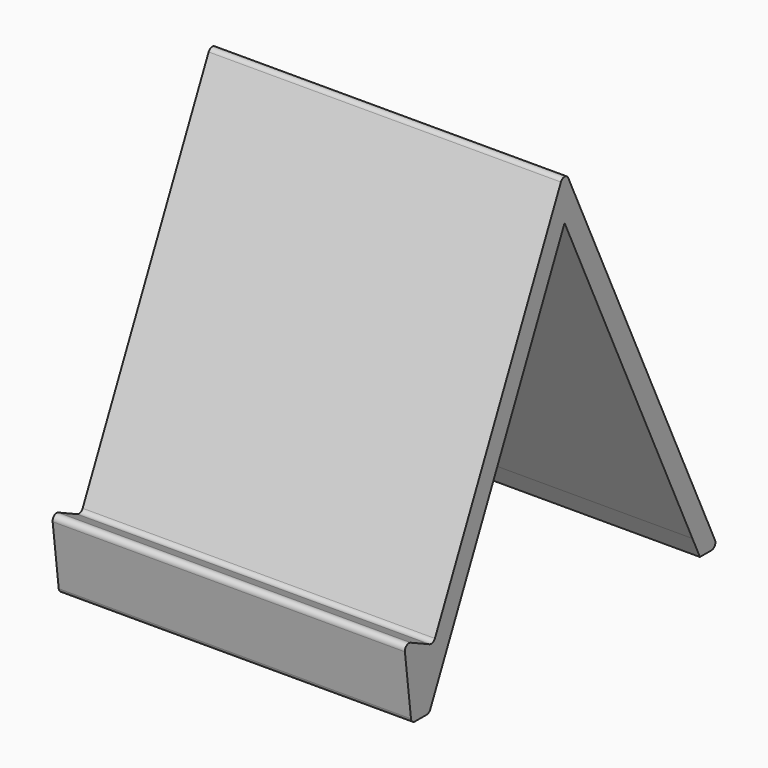
from build123d import *

# Parameters (mm, degrees)
F1_DEPTH = 70
F2_R     = 1


with BuildPart() as f1:
    # F0 (on Right) → F1 (new body)
    with BuildSketch(Plane.YZ):
        Polygon((-1.8379441239, 14.9881287721), (0, 0), (4.4135116758, 0), (6.2787423085, 4), (38.0356435567, 72.1028945007), (69.7925448049, 4), (71.6577754375, 0), (76.0712871133, 0), (38.0356435567, 81.5677008333), (5.4125181724, 11.6071826782), align=None)
    extrude(amount=F1_DEPTH)

    # F2
    f2_edges = [f1.edges().sort_by_distance(p)[0] for p in [
        (35, -1.837944, 14.988129),
        (35, 5.412518, 11.607183),
        (35, 38.035644, 81.567701),
        (35, 0, 0),
        (35, 76.071287, 0),
        (35, 4.413512, 0),
    ]]
    fillet(f2_edges, radius=F2_R)


solid = f1.part
